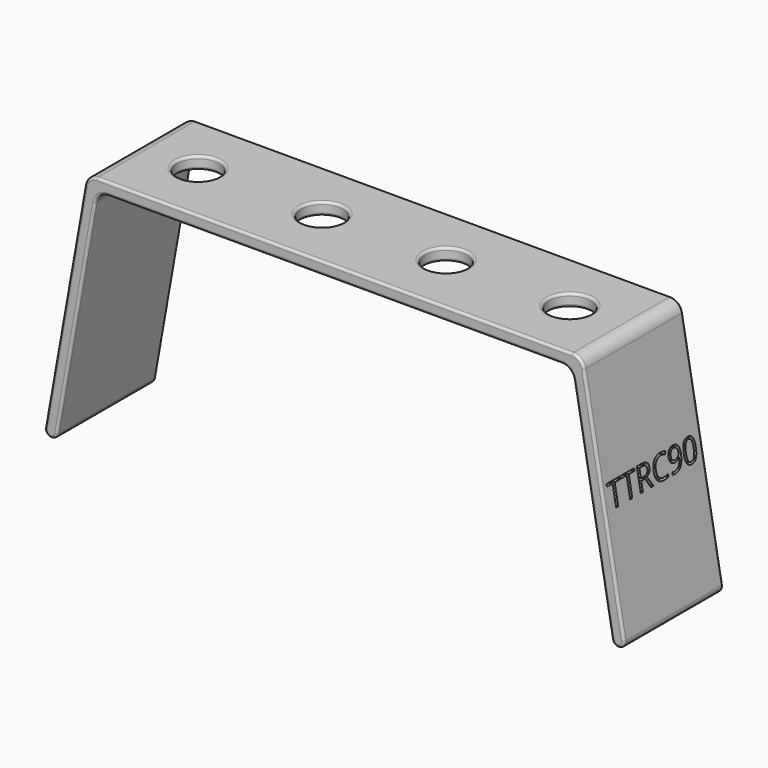
from build123d import *

# Parameters (mm, degrees)
F0_W         = 200
F0_H         = 50
F0_R         = 8.5
F1_DEPTH     = 5
F3_DEPTH     = 50
F4_R         = 5
F5_R         = 2.49999
F6_TEXT_SIZE = 12.8051220488
F7_DEPTH     = 2
F8_TEXT_SIZE = 12.8051220488
F9_DEPTH     = 2
F10_R        = 1
F11_R        = 1


# Not quite as in the source:
# - a fillet or chamfer is up to 0.001 mm smaller than in the source, because OpenCascade refuses the exact size
# - Text() gives the source's letters only with a copy of the font that has no kerning and outlines rounded to 1/6400 em; it was checked with that copy


with BuildPart() as f1:
    # F0 (on Top) → F1 (new body)
    with BuildSketch(Plane.XY):
        Rectangle(F0_W, F0_H)
        with Locations((-75, 0)):
            Circle(F0_R, mode=Mode.SUBTRACT)
        with Locations((-25, 0)):
            Circle(F0_R, mode=Mode.SUBTRACT)
        with Locations((25, 0)):
            Circle(F0_R, mode=Mode.SUBTRACT)
        with Locations((75, 0)):
            Circle(F0_R, mode=Mode.SUBTRACT)
    extrude(amount=F1_DEPTH)

    # F2 (on face) → F3 (join)
    with BuildSketch(Plane.XZ.offset(25)):
        Polygon((-95.8045018441, 0), (-100, 5), (-117.3648177667, -93.4807753012), (-112.2876847073, -93.4807753012), align=None)
        Polygon((117.3648177667, -93.4807753012), (100, 5), (95.8045018441, 0), (112.2876847073, -93.4807753012), align=None)
    extrude(amount=-F3_DEPTH)

    # F4
    f4_edges = [f1.edges().sort_by_distance(p)[0] for p in [
        (95.804502, 0, 0),
        (-95.804502, 0, 0),
        (-100, 0, 5),
        (100, 0, 5),
    ]]
    fillet(f4_edges, radius=F4_R)

    # F5 (radius 2.5 in the source; OpenCascade refuses exactly that, so slightly less here)
    f5_edges = [f1.edges().sort_by_distance(p)[0] for p in [
        (117.364818, 0, -93.480775),
        (112.287685, 0, -93.480775),
        (-112.287685, 0, -93.480775),
        (-117.364818, 0, -93.480775),
    ]]
    fillet(f5_edges, radius=F5_R)

    # F6 (on face) → F7 (cut)
    with BuildSketch(Plane(origin=(-97.8396813976, 0, 17.2517756143), x_dir=(0, -1, 0), z_dir=(-0.984807753, 0, 0.1736481777))):
        with Locations((-22.5, -65.8559650327)):
            Text('TTRC90', F6_TEXT_SIZE, font='Open Sans', text_align=(TextAlign.LEFT, TextAlign.BOTTOM))
    extrude(amount=-F7_DEPTH, mode=Mode.SUBTRACT)

    # F8 (on face) → F9 (cut)
    with BuildSketch(Plane(origin=(97.8396813976, 0, 17.2517756143), x_dir=(0, 1, 0), z_dir=(0.984807753, 0, 0.1736481777))):
        with Locations((-22.5, -65.8559650327)):
            Text('TTRC90', F8_TEXT_SIZE, font='Open Sans', text_align=(TextAlign.LEFT, TextAlign.BOTTOM))
    extrude(amount=-F9_DEPTH, mode=Mode.SUBTRACT)

    # F10
    f10_edges = [f1.edges().sort_by_distance(p)[0] for p in [
        (104.228229, 25, -47.773332),
        (112.778463, 25, -92.895889),
        (94.822942, 25, -1.169778),
        (114.385436, 25, -93.480775),
        (0, 25, 0),
        (116.300549, 25, -92.587748),
        (-94.822942, 25, -1.169778),
        (108.787998, 25, -44.839213),
        (-104.228229, 25, -47.773332),
        (99.01844, 25, 3.830222),
        (-112.778463, 25, -92.895889),
        (0, 25, 5),
        (-114.385436, 25, -93.480775),
        (-99.01844, 25, 3.830222),
        (-116.300549, 25, -92.587748),
        (-108.787998, 25, -44.839213),
        (-104.228229, -25, -47.773332),
        (-112.778463, -25, -92.895889),
        (-94.822942, -25, -1.169778),
        (-114.385436, -25, -93.480775),
        (0, -25, 0),
        (-116.300549, -25, -92.587748),
        (94.822942, -25, -1.169778),
        (-108.787998, -25, -44.839213),
        (104.228229, -25, -47.773332),
        (-99.01844, -25, 3.830222),
        (112.778463, -25, -92.895889),
        (0, -25, 5),
        (114.385436, -25, -93.480775),
        (99.01844, -25, 3.830222),
        (116.300549, -25, -92.587748),
        (108.787998, -25, -44.839213),
    ]]
    fillet(f10_edges, radius=F10_R)

    # F11
    f11_edges = [f1.edges().sort_by_distance(p)[0] for p in [
        (66.5, 0, 5),
        (16.5, 0, 5),
        (-33.5, 0, 5),
        (-83.5, 0, 5),
        (66.5, 0, 0),
        (16.5, 0, 0),
        (-33.5, 0, 0),
        (-83.5, 0, 0),
    ]]
    fillet(f11_edges, radius=F11_R)


solid = f1.part
